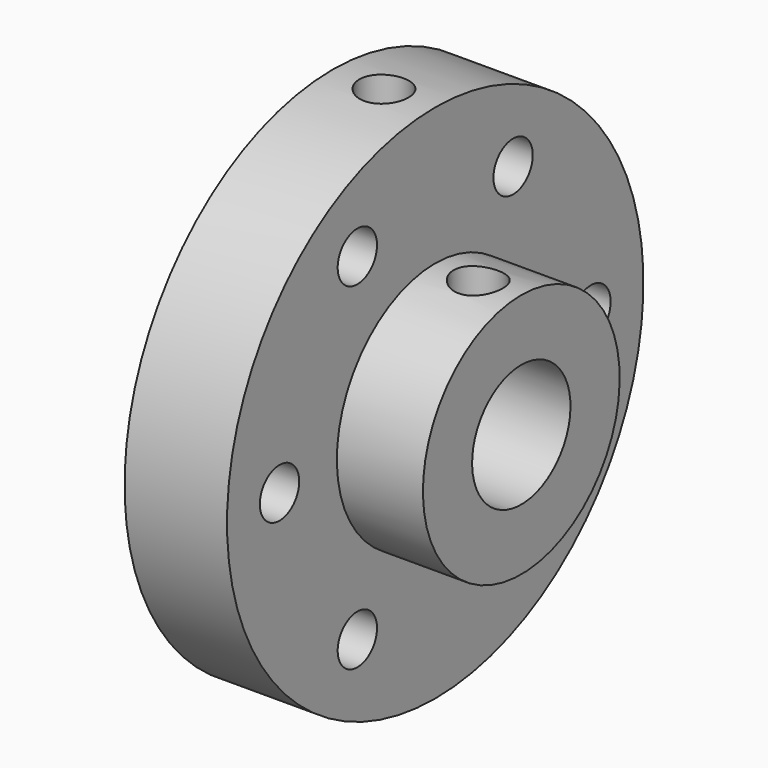
from build123d import *

# Parameters (mm, degrees)
F3_D            = 2.4
F3_COPIES_COUNT = 6
F6_D            = 2.4
F6_DEPTH        = 12.7
F6_START        = 0.0568201
F6_TIP          = 0.7210327428
F9_D            = 2.4
F9_DEPTH        = 5
F9_START        = 0.1212247
F9_TIP          = 0.7210327428


# Not quite as in the source:
# - a pattern or mirror of a feature is missing from the dataset's text; its kind, count and spacing are read off the source's solid


with BuildPart() as f1:
    # F0 (on Front) → F1 (revolve)
    with BuildSketch(Plane.XZ):
        Polygon((-2.5, 12.7), (-2.5, 3), (6.7, 3), (6.7, 6), (2.5, 6), (2.5, 12.7), align=None)
    revolve(axis=Axis((2.1, 0, 0), (1, 0, 0)))

    # F3 (through all)
    with Locations(Plane.YZ.offset(2.5)):
        with Locations((4.75, 8.227241336)):
            f3 = Hole(F3_D / 2)

    # F3_copies: F3 ×6 about axis
    f3_copies_axis = Axis((0, 0, 0), (1, 0, 0))
    for i in range(1, F3_COPIES_COUNT):
        add(f3.rotate(f3_copies_axis, i * 360 / F3_COPIES_COUNT), mode=Mode.SUBTRACT)

    # F6
    # its depths count from where the whole tool has entered the part; down to there all is cleared
    with Locations(Plane.XY.offset(12.7).offset(-F6_START)):
        with Locations((0, 0)):
            Hole(F6_D / 2, depth=F6_DEPTH)
            with Locations((0, 0, -(F6_DEPTH + F6_TIP / 2))):  # 118° drill point
                Cone(0, F6_D / 2, F6_TIP, mode=Mode.SUBTRACT)

    # F9
    # its depths count from where the whole tool has entered the part; down to there all is cleared
    with Locations(Plane.XY.offset(6).offset(-F9_START)):
        with Locations((4.6, 0)):
            Hole(F9_D / 2, depth=F9_DEPTH)
            with Locations((0, 0, -(F9_DEPTH + F9_TIP / 2))):  # 118° drill point
                Cone(0, F9_D / 2, F9_TIP, mode=Mode.SUBTRACT)


solid = f1.part
